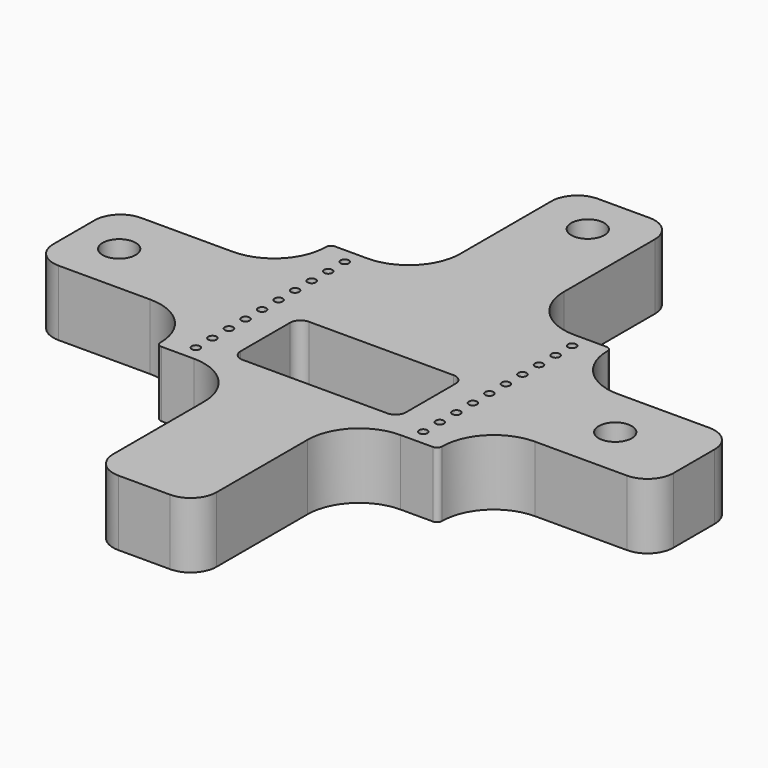
from build123d import *

# Parameters (mm, degrees)
F0_W      = 27.25
F0_H      = 21
F1_DEPTH  = 6.35
F2_R      = 0.4
F3_DEPTH  = 25.4
F5_DEPTH  = 6.35
F6_R      = 1.6
F7_DEPTH  = 25.4
F8_R      = 5
F9_R      = 2.5
F10_R     = 0.49999
F12_DEPTH = 25.4


# Not quite as in the source:
# - a fillet or chamfer is up to 0.001 mm smaller than in the source, because OpenCascade refuses the exact size


with BuildPart() as f1:
    # F0 (on Top) → F1 (new body)
    with BuildSketch(Plane.XY):
        Rectangle(F0_W, F0_H)
    extrude(amount=F1_DEPTH)

    # F2 (on face) → F3 (cut)
    with BuildSketch(Plane.XY.offset(6.35)):
        with Locations((11, 1)):
            Circle(F2_R)
        with Locations((11, 3)):
            Circle(F2_R)
        with Locations((11, 5)):
            Circle(F2_R)
        with Locations((11, 7)):
            Circle(F2_R)
        with Locations((11, 9)):
            Circle(F2_R)
        with Locations((11, -1)):
            Circle(F2_R)
        with Locations((11, -3)):
            Circle(F2_R)
        with Locations((11, -5)):
            Circle(F2_R)
        with Locations((11, -7)):
            Circle(F2_R)
        with Locations((11, -9)):
            Circle(F2_R)
        with Locations((-11, 9)):
            Circle(F2_R)
        with Locations((-11, 7)):
            Circle(F2_R)
        with Locations((-11, 5)):
            Circle(F2_R)
        with Locations((-11, 3)):
            Circle(F2_R)
        with Locations((-11, 1)):
            Circle(F2_R)
        with Locations((-11, -1)):
            Circle(F2_R)
        with Locations((-11, -3)):
            Circle(F2_R)
        with Locations((-11, -5)):
            Circle(F2_R)
        with Locations((-11, -7)):
            Circle(F2_R)
        with Locations((-11, -9)):
            Circle(F2_R)
    extrude(amount=-F3_DEPTH, mode=Mode.SUBTRACT)

    # F4 (on face) → F5 (join)
    with BuildSketch(Plane.XY.offset(6.35)):
        Polygon((5, 29), (0, 29), (-5, 29), (-5, 10.5), (0, 10.5), (5, 10.5), align=None)
        Polygon((-5, -10.5), (-5, -29), (0, -29), (5, -29), (5, -10.5), (0, -10.5), align=None)
        Polygon((-30, 5), (-30, 0), (-30, -5), (-13.625, -5), (-13.625, 0), (-13.625, 5), align=None)
        Polygon((30, 5), (13.625, 5), (13.625, 0), (13.625, -5), (30, -5), (30, 0), align=None)
    extrude(amount=-F5_DEPTH)

    # F6 (on face) → F7 (cut)
    with BuildSketch(Plane.XY.offset(6.35)):
        with Locations((-25.625, 0)):
            Circle(F6_R)
        with Locations((22.375, 0)):
            Circle(F6_R)
        with Locations((0, 24.65)):
            Circle(F6_R)
    extrude(amount=-F7_DEPTH, mode=Mode.SUBTRACT)

    # F8
    f8_edges = [f1.edges().sort_by_distance(p)[0] for p in [
        (-5, 10.5, 3.175),
        (-13.625, 5, 3.175),
        (-13.625, -5, 3.175),
        (-5, -10.5, 3.175),
        (5, 10.5, 3.175),
        (13.625, 5, 3.175),
        (13.625, -5, 3.175),
        (5, -10.5, 3.175),
    ]]
    fillet(f8_edges, radius=F8_R)

    # F9
    f9_edges = [f1.edges().sort_by_distance(p)[0] for p in [
        (-30, 5, 3.175),
        (-5, 29, 3.175),
        (5, 29, 3.175),
        (-30, -5, 3.175),
        (-5, -29, 3.175),
        (5, -29, 3.175),
        (30, 5, 3.175),
        (30, -5, 3.175),
    ]]
    fillet(f9_edges, radius=F9_R)

    # F10 (radius 0.5 in the source; OpenCascade refuses exactly that, so slightly less here)
    f10_edges = [f1.edges().sort_by_distance(p)[0] for p in [
        (-13.625, -10.5, 3.175),
        (13.625, -10.5, 3.175),
        (-13.625, 10.5, 3.175),
        (13.625, 10.5, 3.175),
    ]]
    fillet(f10_edges, radius=F10_R)

    # F11 (on face) → F12 (cut)
    with BuildSketch(Plane.XY.offset(6.35)):
        with BuildLine():
            Line((7, -0.35), (-7, -0.35))
            ThreePointArc((-7, -0.35), (-7.7071067812, -0.6428932188), (-8, -1.35))
            Line((-8, -1.35), (-8, -7.35))
            ThreePointArc((-8, -7.35), (-7.7071067812, -8.0571067812), (-7, -8.35))
            Line((-7, -8.35), (7, -8.35))
            ThreePointArc((7, -8.35), (7.7071067812, -8.0571067812), (8, -7.35))
            Line((8, -7.35), (8, -1.35))
            ThreePointArc((8, -1.35), (7.7071067812, -0.6428932188), (7, -0.35))
        make_face()
    extrude(amount=-F12_DEPTH, mode=Mode.SUBTRACT)


solid = f1.part
